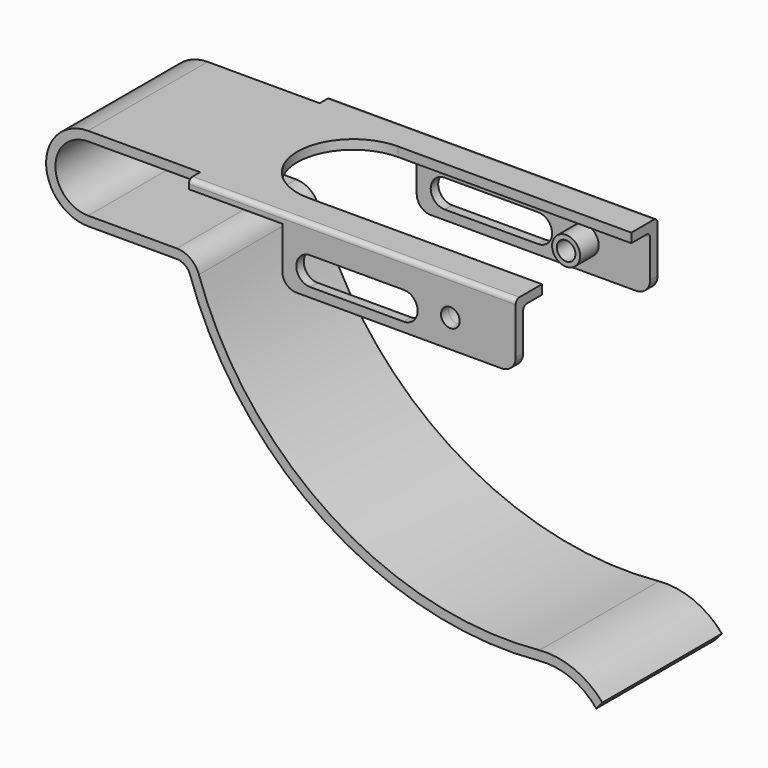
from build123d import *

# Parameters (mm, degrees)
F1_DEPTH  = 16
F2_W      = 70
F2_H      = 3
F3_DEPTH  = 2
F4_W      = 50
F4_H      = 14
F5_DEPTH  = 2
F6_R      = 1
F9_DEPTH  = 2
F11_DEPTH = 38.001
F13_D     = 4
F14_R     = 3
F14_R_2   = 2
F15_DEPTH = 5
F16_R     = 3


# Not quite as in the source:
# - a pattern or mirror of a feature is missing from the dataset's text; its kind, count and spacing are read off the source's solid


with BuildPart() as f1:
    # F0 (on Front) → F1 (new body)
    with BuildSketch(Plane.XZ):
        with BuildLine():
            Line((94, 9), (0, 9))
            ThreePointArc((0, 9), (-9, 0), (0, -9))
            Line((0, -9), (19, -9))
            ThreePointArc((19, -9), (20.7464347921, -9.5607448848), (21.84, -11.0333563221))
            ThreePointArc((21.84, -11.0333563221), (50.8304964021, -48.2470687705), (96.6350861079, -59.5275314258))
            ThreePointArc((96.6350861079, -59.5275314258), (103.3892729035, -60.5026852737), (108.8800565509, -64.5550005668))
            Line((108.8800565509, -64.5550005668), (110.184856953, -63))
            ThreePointArc((110.184856953, -63), (104.1026052212, -58.6336361635), (96.6997621323, -57.5125503141))
            ThreePointArc((96.6997621323, -57.5125503141), (52.0235205329, -46.636858721), (23.7333333333, -10.3889272035))
            ThreePointArc((23.7333333333, -10.3889272035), (21.9107246536, -7.9345748081), (19, -7))
            Line((19, -7), (0, -7))
            ThreePointArc((0, -7), (-7, 0), (0, 7))
            Line((0, 7), (94, 7))
            Line((94, 7), (94, 9))
        make_face()
    extrude(amount=F1_DEPTH)

    # F2 (on face) → F3 (join)
    with BuildSketch(Plane.XY.offset(9)):
        with Locations((59, -17.5)):
            Rectangle(F2_W, F2_H)
    extrude(amount=-F3_DEPTH)

    # F4 (on face) → F5 (join)
    with BuildSketch(Plane.XZ.offset(19)):
        with Locations((69, 2)):
            Rectangle(F4_W, F4_H)
    extrude(amount=-F5_DEPTH)

    # F6
    f6_edges = [f1.edges().sort_by_distance(p)[0] for p in [
        (59, -19, 9),
        (69, -17, 7),
    ]]
    fillet(f6_edges, radius=F6_R)

    # F7: F1 across plane


with BuildPart() as f1_1:
    add(f1.part)
    add(f1.part.mirror(Plane.XZ))

    # F8 (on face) → F9 (cut)
    with BuildSketch(Plane.XY.offset(9)):
        with BuildLine():
            Line((94, 11.9645609066), (44, 11.9645609066))
            ThreePointArc((44, 11.9645609066), (32.0354390934, 0), (44, -11.9645609066))
            Line((44, -11.9645609066), (94, -11.9645609066))
            Line((94, -11.9645609066), (94, 11.9645609066))
        make_face()
    extrude(amount=-F9_DEPTH, mode=Mode.SUBTRACT)

    # F10 (on face) → F11 (cut, through all)
    with BuildSketch(Plane.XZ.offset(19)):
        with BuildLine():
            ThreePointArc((50, 3), (47, 0), (50, -3))
            Line((50, -3), (70, -3))
            ThreePointArc((70, -3), (73, 0), (70, 3))
            Line((70, 3), (50, 3))
        make_face()
    extrude(amount=-F11_DEPTH, mode=Mode.SUBTRACT)

    # F13 (through all)
    with Locations(Plane.XZ.offset(19)):
        with Locations((80, 1)):
            Hole(F13_D / 2)

    # F14 (on face) → F15 (join)
    with BuildSketch(Plane(origin=(0, -17, 0), x_dir=(-1, 0, 0), z_dir=(0, 1, 0))):
        with Locations((-80, 1)):
            Circle(F14_R)
        with Locations((-80, 1)):
            Circle(F14_R_2, mode=Mode.SUBTRACT)
    f15 = extrude(amount=F15_DEPTH)

    # F15_copies: F15 across plane
    add(f15.mirror(Plane.ZX))

    # F16
    f16_edges = [f1_1.edges().sort_by_distance(p)[0] for p in [
        (94, 18, -5),
        (94, -18, -5),
        (44, -18, -5),
        (44, 18, -5),
    ]]
    fillet(f16_edges, radius=F16_R)


solid = f1_1.part
